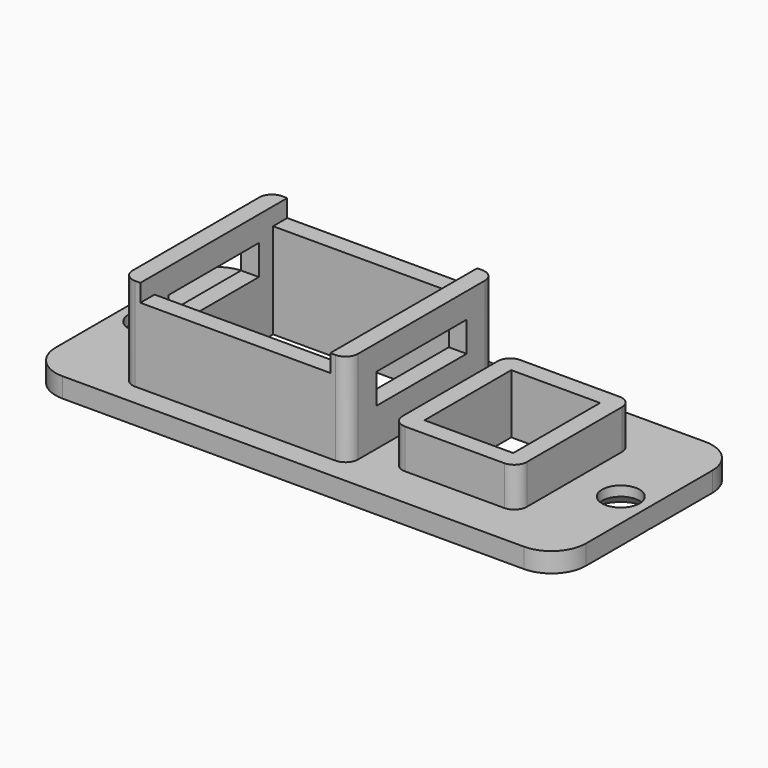
from build123d import *

# Parameters (mm, degrees)
F1_DEPTH  = 2
F2_R      = 1.9
F3_DEPTH  = 2.001
F5_W      = 19.2532
F5_H      = 15.0114
F6_DEPTH  = 2.001
F7_W      = 19.2532
F7_H      = 15.0114
F8_DEPTH  = 9.43
F9_W      = 11.43
F9_H      = 3.048
F10_DEPTH = 45.9292
F11_W     = 19.2532
F11_H     = 18.6114
F12_DEPTH = 1.778
F13_W     = 2.7532
F13_H     = 15.0114
F14_DEPTH = 2
F15_SIZE  = 1.8
F16_W     = 9
F16_H     = 11
F17_DEPTH = 2.001
F18_W     = 9
F18_H     = 11
F19_DEPTH = 4


# Not quite as in the source:
# - a fillet or chamfer that OpenCascade refuses, or shapes differently, is made with other operations: its cross-section is extruded or revolved along the edge and cut away or added


with BuildPart() as f1:
    # F0 (on Top) → F1 (new body)
    with BuildSketch(Plane.XY):
        with BuildLine():
            ThreePointArc((26.875, 8), (25.8498737342, 10.4748737342), (23.375, 11.5))
            Line((23.375, 11.5), (-23.375, 11.5))
            ThreePointArc((-23.375, 11.5), (-25.8498737342, 10.4748737342), (-26.875, 8))
            Line((-26.875, 8), (-26.875, -8))
            ThreePointArc((-26.875, -8), (-25.8498737342, -10.4748737342), (-23.375, -11.5))
            Line((-23.375, -11.5), (23.375, -11.5))
            ThreePointArc((23.375, -11.5), (25.8498737342, -10.4748737342), (26.875, -8))
            Line((26.875, -8), (26.875, 8))
        make_face()
    extrude(amount=F1_DEPTH)

    # F2 (on face) → F3 (cut, through all)
    with BuildSketch(Plane.XY.offset(2)):
        with Locations((-24, 0)):
            Circle(F2_R)
        with Locations((24, 0)):
            Circle(F2_R)
    extrude(amount=-F3_DEPTH, mode=Mode.SUBTRACT)

    # F4: chamfer of 1 on 2 edges, made by hand

    # F4_s1 → F4_t2 (revolve, cut)
    with BuildSketch(Plane.XZ):
        Polygon((-21.1, 0), (-22.1, 1), (-22.1, 0), align=None)
    revolve(axis=Axis((-24, 0, 0), (0, 0, 1)), mode=Mode.SUBTRACT)

    # F4_s3 → F4_t4 (revolve, cut)
    with BuildSketch(Plane.XZ):
        Polygon((26.9, 0), (25.9, 1), (25.9, 0), align=None)
    revolve(axis=Axis((24, 0, 0), (0, 0, 1)), mode=Mode.SUBTRACT)

    # F5 (on face) → F6 (cut, through all)
    with BuildSketch(Plane.XY.offset(2)):
        with Locations((-7.6266, 0)):
            Rectangle(F5_W, F5_H)
    extrude(amount=-F6_DEPTH, mode=Mode.SUBTRACT)

    # F7 (on face) → F8 (join)
    with BuildSketch(Plane.XY.offset(2)):
        with BuildLine():
            ThreePointArc((3.8, 8.0357), (3.4280256121, 8.9337256121), (2.53, 9.3057))
            Line((2.53, 9.3057), (-17.7832, 9.3057))
            ThreePointArc((-17.7832, 9.3057), (-18.6812256121, 8.9337256121), (-19.0532, 8.0357))
            Line((-19.0532, 8.0357), (-19.0532, -8.0357))
            ThreePointArc((-19.0532, -8.0357), (-18.6812256121, -8.9337256121), (-17.7832, -9.3057))
            Line((-17.7832, -9.3057), (2.53, -9.3057))
            ThreePointArc((2.53, -9.3057), (3.4280256121, -8.9337256121), (3.8, -8.0357))
            Line((3.8, -8.0357), (3.8, 8.0357))
        make_face()
        with Locations((-7.6266, 0)):
            Rectangle(F7_W, F7_H, mode=Mode.SUBTRACT)
    extrude(amount=F8_DEPTH)

    # F9 (on face) → F10 (cut, through all)
    with BuildSketch(Plane(origin=(-19.0532, 0, 0), x_dir=(0, -1, 0), z_dir=(-1, 0, 0))):
        with Locations((0, 7.366)):
            Rectangle(F9_W, F9_H)
    extrude(amount=-F10_DEPTH, mode=Mode.SUBTRACT)

    # F11 (on face) → F12 (cut)
    with BuildSketch(Plane.XY.offset(11.43)):
        with Locations((-7.6266, 0)):
            Rectangle(F11_W, F11_H)
    extrude(amount=-F12_DEPTH, mode=Mode.SUBTRACT)

    # F13 (on face) → F14 (join)
    with BuildSketch(Plane(origin=(0, 0, 0), x_dir=(1, 0, 0), z_dir=(0, 0, -1))):
        with Locations((0.6234, 0)):
            Rectangle(F13_W, F13_H)
    extrude(amount=-F14_DEPTH)

    # F15
    f15_edges = [f1.edges().sort_by_distance(p)[0] for p in [
        (-0.7532, 0, 2),
    ]]
    chamfer(f15_edges, length=F15_SIZE)

    # F16 (on face) → F17 (cut, through all)
    with BuildSketch(Plane.XY.offset(2)):
        with Locations((13, 0)):
            Rectangle(F16_W, F16_H)
    extrude(amount=-F17_DEPTH, mode=Mode.SUBTRACT)

    # F18 (on face) → F19 (join)
    with BuildSketch(Plane.XY.offset(2)):
        with BuildLine():
            ThreePointArc((18.03, -7.3), (18.9280256121, -6.9280256121), (19.3, -6.03))
            Line((19.3, -6.03), (19.3, 6.03))
            ThreePointArc((19.3, 6.03), (18.9280256121, 6.9280256121), (18.03, 7.3))
            Line((18.03, 7.3), (7.97, 7.3))
            ThreePointArc((7.97, 7.3), (7.0719743879, 6.9280256121), (6.7, 6.03))
            Line((6.7, 6.03), (6.7, -6.03))
            ThreePointArc((6.7, -6.03), (7.0719743879, -6.9280256121), (7.97, -7.3))
            Line((7.97, -7.3), (18.03, -7.3))
        make_face()
        with Locations((13, 0)):
            Rectangle(F18_W, F18_H, mode=Mode.SUBTRACT)
    extrude(amount=F19_DEPTH)


solid = f1.part
